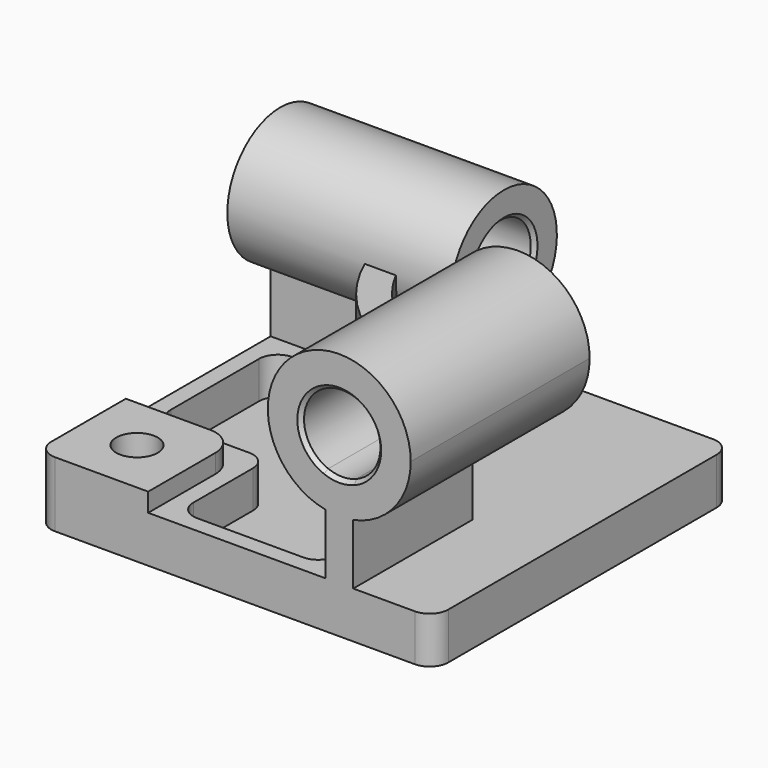
from build123d import *

# Parameters (mm, degrees)
F0_W            = 213
F0_H            = 200
F1_DEPTH        = 25
F2_W            = 60
F2_H            = 60
F3_DEPTH        = 10
F4_R            = 10
F5_R            = 15
F6_DEPTH        = 20
F7_DEPTH        = 70
F8_R            = 10
F10_DEPTH       = 120
F11_DEPTH       = 120
F12_SIZE        = 2
F14_DEPTH       = 120
F15_DEPTH       = 120
F16_SIZE        = 2
F18_D           = 14.75
F18_CBORE_D     = 22.25
F18_CBORE_DEPTH = 14
F19_SIZE        = 2
F20_SIZE        = 2


with BuildPart() as f1:
    # F0 (on Top) → F1 (new body)
    with BuildSketch(Plane.XY):
        Rectangle(F0_W, F0_H)
    extrude(amount=F1_DEPTH)

    # F2 (on face) → F3 (join)
    with BuildSketch(Plane.XY.offset(25)):
        with Locations((-76.5, -70)):
            Rectangle(F2_W, F2_H)
    extrude(amount=F3_DEPTH)

    # F4
    f4_edges = [f1.edges().sort_by_distance(p)[0] for p in [
        (-106.5, -100, 17.5),
        (106.5, -100, 12.5),
        (106.5, 100, 12.5),
        (-106.5, 100, 12.5),
    ]]
    fillet(f4_edges, radius=F4_R)

    # F5
    f5_edges = [f1.edges().sort_by_distance(p)[0] for p in [
        (-46.5, -40, 30),
    ]]
    fillet(f5_edges, radius=F5_R)

    # F2 (on face) → F6 (cut)
    with BuildSketch(Plane.XY.offset(25)):
        with BuildLine():
            Line((-48.3758740693, 48.0959181604), (-97.5, 48.0959181604))
            Line((-97.5, 48.0959181604), (-97.5, -31))
            Line((-97.5, -31), (-37.5, -31))
            Line((-37.5, -31), (-37.5, -91))
            Line((-37.5, -91), (39.5, -91))
            Line((39.5, -91), (39.5, -41.445053726))
            ThreePointArc((39.5, -41.445053726), (-17.8631347732, -9.8501114582), (-48.3758740693, 48.0959181604))
        make_face()
    extrude(amount=-F6_DEPTH, mode=Mode.SUBTRACT)

    # F2 (on face) → F7 (join)
    with BuildSketch(Plane.XY.offset(25)):
        with BuildLine():
            Line((48.5, -33.9230484541), (48.5, -100))
            Line((48.5, -100), (63.5, -100))
            Line((63.5, -100), (63.5, -20))
            ThreePointArc((63.5, -20), (-0.1396103068, 6.3603896932), (-26.5, 70))
            Line((-26.5, 70), (-106.5, 70))
            Line((-106.5, 70), (-106.5, 57.0959181604))
            Line((-106.5, 57.0959181604), (-40.7040530492, 57.0959181604))
            ThreePointArc((-40.7040530492, 57.0959181604), (-11.4900969244, -3.4947982055), (48.5, -33.9230484541))
        make_face()
    extrude(amount=F7_DEPTH)

    # F8
    f8_edges = [f1.edges().sort_by_distance(p)[0] for p in [
        (-48.375874, 48.095918, 15),
        (39.5, -41.445054, 15),
        (-37.5, -31, 15),
        (-97.5, 48.095918, 15),
        (39.5, -91, 15),
        (-37.5, -91, 15),
        (-97.5, -31, 15),
    ]]
    fillet(f8_edges, radius=F8_R)

    # F9 (on face) → F10 (cut)
    with BuildSketch(Plane(origin=(-106.5, 0, 0), x_dir=(0, -1, 0), z_dir=(-1, 0, 0))):
        with BuildLine():
            ThreePointArc((-43.0479590802, 95), (-75.5476082656, 111.621023417), (-70, 75.5418097458))
            Line((-70, 75.5418097458), (-70, 95))
            Line((-70, 95), (-57.0959181604, 95))
            Line((-57.0959181604, 95), (-57.0959181604, 75.5418097458))
            ThreePointArc((-57.0959181604, 75.5418097458), (-46.9269356632, 83.0003508146), (-43.0479590802, 95))
        make_face()
        with BuildLine():
            Line((-70, 95), (-70, 75.5418097458))
            ThreePointArc((-70, 75.5418097458), (-63.5479590802, 74.5), (-57.0959181604, 75.5418097458))
            Line((-57.0959181604, 75.5418097458), (-57.0959181604, 95))
            Line((-57.0959181604, 95), (-70, 95))
        make_face()
        with BuildLine():
            ThreePointArc((-57.0959181604, 60.09124511), (-36.2597065468, 72.2931447868), (-28.0479590802, 95))
            ThreePointArc((-28.0479590802, 95), (-86.2548142934, 122.2882525334), (-70, 60.09124511))
            Line((-70, 60.09124511), (-70, 75.5418097458))
            ThreePointArc((-70, 75.5418097458), (-75.5476082656, 111.621023417), (-43.0479590802, 95))
            ThreePointArc((-43.0479590802, 95), (-46.9269356632, 83.0003508146), (-57.0959181604, 75.5418097458))
            Line((-57.0959181604, 75.5418097458), (-57.0959181604, 60.09124511))
        make_face()
    extrude(amount=-F10_DEPTH, mode=Mode.SUBTRACT)

    # F9 (on face) → F11 (join)
    with BuildSketch(Plane(origin=(-106.5, 0, 0), x_dir=(0, -1, 0), z_dir=(-1, 0, 0))):
        with BuildLine():
            ThreePointArc((-57.0959181604, 60.09124511), (-36.2597065468, 72.2931447868), (-28.0479590802, 95))
            ThreePointArc((-28.0479590802, 95), (-86.2548142934, 122.2882525334), (-70, 60.09124511))
            Line((-70, 60.09124511), (-70, 75.5418097458))
            ThreePointArc((-70, 75.5418097458), (-75.5476082656, 111.621023417), (-43.0479590802, 95))
            ThreePointArc((-43.0479590802, 95), (-46.9269356632, 83.0003508146), (-57.0959181604, 75.5418097458))
            Line((-57.0959181604, 75.5418097458), (-57.0959181604, 60.09124511))
        make_face()
        with BuildLine():
            Line((-70, 75.5418097458), (-70, 60.09124511))
            ThreePointArc((-70, 60.09124511), (-63.5479590802, 59.5), (-57.0959181604, 60.09124511))
            Line((-57.0959181604, 60.09124511), (-57.0959181604, 75.5418097458))
            ThreePointArc((-57.0959181604, 75.5418097458), (-63.5479590802, 74.5), (-70, 75.5418097458))
        make_face()
    extrude(amount=-F11_DEPTH)

    # F12
    f12_edges = [f1.edges().sort_by_distance(p)[0] for p in [
        (-106.5, 84.047959, 95),
    ]]
    chamfer(f12_edges, length=F12_SIZE)

    # F13 (on face) → F14 (cut)
    with BuildSketch(Plane.XZ.offset(100)):
        with BuildLine():
            ThreePointArc((76.5, 95), (44.4566036194, 111.9410743461), (48.5, 75.9212159717))
            Line((48.5, 75.9212159717), (48.5, 95))
            Line((48.5, 95), (63.5, 95))
            Line((63.5, 95), (63.5, 75.9212159717))
            ThreePointArc((63.5, 75.9212159717), (72.9410743461, 83.4566036194), (76.5, 95))
        make_face()
        with BuildLine():
            Line((48.5, 95), (48.5, 75.9212159717))
            ThreePointArc((48.5, 75.9212159717), (56, 74.5), (63.5, 75.9212159717))
            Line((63.5, 75.9212159717), (63.5, 95))
            Line((63.5, 95), (48.5, 95))
        make_face()
    extrude(amount=-F14_DEPTH, mode=Mode.SUBTRACT)

    # F13 (on face) → F15 (join)
    with BuildSketch(Plane.XZ.offset(100)):
        with BuildLine():
            ThreePointArc((63.5, 57.4073514866), (85.6391503948, 70.6899612068), (94.3335, 95))
            ThreePointArc((94.3335, 95), (31.6899612068, 124.6391503948), (48.5, 57.4073514866))
            Line((48.5, 57.4073514866), (48.5, 75.9212159717))
            ThreePointArc((48.5, 75.9212159717), (44.4566036194, 111.9410743461), (76.5, 95))
            ThreePointArc((76.5, 95), (72.9410743461, 83.4566036194), (63.5, 75.9212159717))
            Line((63.5, 75.9212159717), (63.5, 57.4073514866))
        make_face()
        with BuildLine():
            Line((48.5, 75.9212159717), (48.5, 57.4073514866))
            ThreePointArc((48.5, 57.4073514866), (56, 56.6665), (63.5, 57.4073514866))
            Line((63.5, 57.4073514866), (63.5, 75.9212159717))
            ThreePointArc((63.5, 75.9212159717), (56, 74.5), (48.5, 75.9212159717))
        make_face()
    extrude(amount=-F15_DEPTH)

    # F16
    f16_edges = [f1.edges().sort_by_distance(p)[0] for p in [
        (35.5, -100, 95),
    ]]
    chamfer(f16_edges, length=F16_SIZE)

    # F18 (through all)
    with Locations(Plane.XY.offset(35)):
        with Locations((-76.5, -70)):
            CounterBoreHole(F18_D / 2, F18_CBORE_D / 2, F18_CBORE_DEPTH)

    # F19
    f19_edges = [f1.edges().sort_by_distance(p)[0] for p in [
        (35.5, 20, 95),
    ]]
    chamfer(f19_edges, length=F19_SIZE)

    # F20
    f20_edges = [f1.edges().sort_by_distance(p)[0] for p in [
        (13.5, 84.047959, 95),
    ]]
    chamfer(f20_edges, length=F20_SIZE)


solid = f1.part
